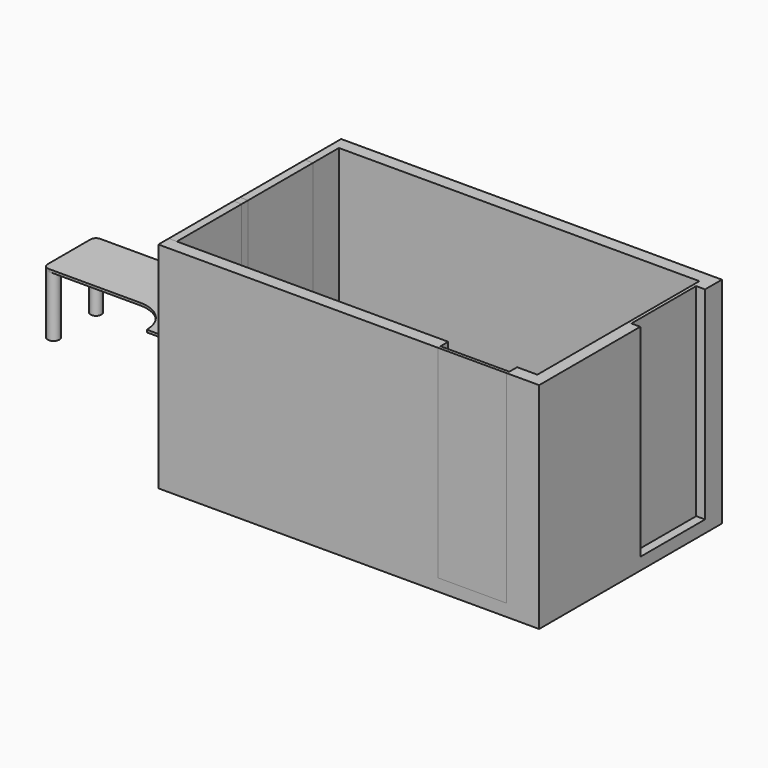
from build123d import *

# Parameters (mm, degrees)
F0_W      = 100
F0_H      = 1000
F0_H_2    = 100
F0_W_2    = 850
F0_H_3    = 120
F0_H_4    = 40
F0_W_3    = 110
F0_W_4    = 40
F1_DEPTH  = 150
F2_DEPTH  = 150
F3_DEPTH  = 2500
F4_DEPTH  = 2500
F5_DEPTH  = 2500
F8_DEPTH  = 15
F9_DEPTH  = 760
F11_W     = 1600
F11_H     = 430
F12_DEPTH = 900
F13_W     = 390
F13_H     = 1450
F14_DEPTH = 770
F15_W     = 322.5
F15_H     = 336
F16_DEPTH = 390
F17_R     = 300
F18_DEPTH = 80
F19_R     = 40
F20_DEPTH = 400
F21_W     = 440
F21_H     = 400
F21_W_2   = 60
F22_DEPTH = 60
F23_DEPTH = 600
F24_R     = 50
F25_SIZE  = 40


with BuildPart() as f1:
    # F0 (on Top) → F1 (new body)
    with BuildSketch(Plane.XY):
        Polygon((300, 2500), (300, 0), (3350, 0), (4200, 0), (4450, 0), (4450, 1400), (4450, 2400), (4450, 2500), align=None)
        Polygon((0, 2500), (300, 2500), (4450, 2500), (4450, 2400), (4490, 2400), (4600, 2400), (4600, 2660), (-100, 2660), (-100, 2100), (0, 2100), align=None)
        with Locations((-50, 1600)):
            Rectangle(F0_W, F0_H)
        with Locations((-50, 1050)):
            Rectangle(F0_W, F0_H_2)
        with Locations((-50, 500)):
            Rectangle(F0_W, F0_H)
        Polygon((300, 0), (0, 0), (-100, 0), (-100, -160), (3350, -160), (3350, -120), (3350, 0), align=None)
        with Locations((3775, -60)):
            Rectangle(F0_W_2, F0_H_3)
        with Locations((3775, -140)):
            Rectangle(F0_W_2, F0_H_4)
        Polygon((4450, 0), (4200, 0), (4200, -120), (4200, -160), (4600, -160), (4600, 1400), (4490, 1400), (4450, 1400), align=None)
        with Locations((4545, 1900)):
            Rectangle(F0_W_3, F0_H)
        with Locations((4470, 1900)):
            Rectangle(F0_W_4, F0_H)
    extrude(amount=-F1_DEPTH)

    # F0 (on Top) → F2 (join, through all)
    with BuildSketch(Plane.XY):
        Polygon((0, 1000), (0, 0), (300, 0), (300, 2500), (0, 2500), (0, 2100), (0, 1100), align=None)
    extrude(amount=-F2_DEPTH)

    # F0 (on Top) → F3 (join)
    with BuildSketch(Plane.XY):
        Polygon((0, 2500), (300, 2500), (4450, 2500), (4450, 2400), (4490, 2400), (4600, 2400), (4600, 2660), (-100, 2660), (-100, 2100), (0, 2100), align=None)
        Polygon((4450, 0), (4200, 0), (4200, -120), (4200, -160), (4600, -160), (4600, 1400), (4490, 1400), (4450, 1400), align=None)
        Polygon((300, 0), (0, 0), (-100, 0), (-100, -160), (3350, -160), (3350, -120), (3350, 0), align=None)
        with Locations((-50, 1050)):
            Rectangle(F0_W, F0_H_2)
    extrude(amount=F3_DEPTH)


with BuildPart() as f4:
    # F0 (on Top) → F4 (new body, through all)
    with BuildSketch(Plane.XY):
        with Locations((-50, 1600)):
            Rectangle(F0_W, F0_H)
    extrude(amount=F4_DEPTH)


with BuildPart() as f4b:
    # F0 (on Top) → F4, piece 2 (new body, through all)
    with BuildSketch(Plane.XY):
        with Locations((-50, 500)):
            Rectangle(F0_W, F0_H)
    extrude(amount=F4_DEPTH)


with BuildPart() as f5:
    # F0 (on Top) → F5 (new body, through all)
    with BuildSketch(Plane.XY):
        with Locations((4470, 1900)):
            Rectangle(F0_W_4, F0_H)
    extrude(amount=F5_DEPTH)


with BuildPart() as f5b:
    # F0 (on Top) → F5, piece 2 (new body, through all)
    with BuildSketch(Plane.XY):
        with Locations((3775, -140)):
            Rectangle(F0_W_2, F0_H_4)
    extrude(amount=F5_DEPTH)


with BuildPart() as f8:
    # F7 (on offset) → F8 (new body, symmetric)
    with BuildSketch(Plane.XY.offset(760)):
        with BuildLine():
            Line((2680.377719402, 2169.4638956216), (646.4488137391, 2169.4638956216))
            ThreePointArc((646.4488137391, 2169.4638956216), (688.5376842462, 2152.0301146325), (705.9714652353, 2109.9412441254))
            ThreePointArc((705.9714652353, 2109.9412441254), (646.4488137391, 2050.4185926292), (586.9261622429, 2109.9412441254))
            Line((586.9261622429, 2109.9412441254), (586.9261622429, 1040.2058445736))
            ThreePointArc((586.9261622429, 1040.2058445736), (657.6681111949, 1110.9477935256), (728.410060147, 1040.2058445736))
            ThreePointArc((728.410060147, 1040.2058445736), (707.6902230133, 990.1837327553), (657.6681111949, 969.4638956216))
            Line((657.6681111949, 969.4638956216), (1146.9261622429, 969.4638956216))
            ThreePointArc((1146.9261622429, 969.4638956216), (1264.0834497683, 1252.3066080962), (1546.9261622429, 1369.4638956216))
            Line((1546.9261622429, 1369.4638956216), (2675.2513630672, 1369.4638956216))
            ThreePointArc((2675.2513630672, 1369.4638956216), (2624.5696265299, 1491.8204313346), (2746.9261622429, 1441.1386947972))
            Line((2746.9261622429, 1441.1386947972), (2746.9261622429, 2102.9154527807))
            ThreePointArc((2746.9261622429, 2102.9154527807), (2633.3208641919, 2055.8585975705), (2680.377719402, 2169.4638956216))
        make_face()
        with BuildLine():
            ThreePointArc((705.9714652353, 2109.9412441254), (688.5376842462, 2152.0301146325), (646.4488137391, 2169.4638956216))
            ThreePointArc((646.4488137391, 2169.4638956216), (604.3599432319, 2152.0301146325), (586.9261622429, 2109.9412441254))
            ThreePointArc((586.9261622429, 2109.9412441254), (646.4488137391, 2050.4185926292), (705.9714652353, 2109.9412441254))
        make_face()
        with BuildLine():
            ThreePointArc((2746.9261622429, 2102.9154527807), (2727.4345746122, 2149.9723079909), (2680.377719402, 2169.4638956216))
            ThreePointArc((2680.377719402, 2169.4638956216), (2633.3208641919, 2055.8585975705), (2746.9261622429, 2102.9154527807))
        make_face()
        with BuildLine():
            ThreePointArc((2675.2513630672, 1369.4638956216), (2725.9330996045, 1390.4569582599), (2746.9261622429, 1441.1386947972))
            ThreePointArc((2746.9261622429, 1441.1386947972), (2624.5696265299, 1491.8204313346), (2675.2513630672, 1369.4638956216))
        make_face()
        with BuildLine():
            ThreePointArc((728.410060147, 1040.2058445736), (657.6681111949, 1110.9477935256), (586.9261622429, 1040.2058445736))
            ThreePointArc((586.9261622429, 1040.2058445736), (607.6459993766, 990.1837327553), (657.6681111949, 969.4638956216))
            ThreePointArc((657.6681111949, 969.4638956216), (707.6902230133, 990.1837327553), (728.410060147, 1040.2058445736))
        make_face()
    extrude(amount=F8_DEPTH, both=True)

    # F7 (on offset) → F9 (join, through all)
    with BuildSketch(Plane.XY.offset(760)):
        with BuildLine():
            ThreePointArc((705.9714652353, 2109.9412441254), (688.5376842462, 2152.0301146325), (646.4488137391, 2169.4638956216))
            ThreePointArc((646.4488137391, 2169.4638956216), (604.3599432319, 2152.0301146325), (586.9261622429, 2109.9412441254))
            ThreePointArc((586.9261622429, 2109.9412441254), (646.4488137391, 2050.4185926292), (705.9714652353, 2109.9412441254))
        make_face()
        with BuildLine():
            ThreePointArc((2746.9261622429, 2102.9154527807), (2727.4345746122, 2149.9723079909), (2680.377719402, 2169.4638956216))
            ThreePointArc((2680.377719402, 2169.4638956216), (2633.3208641919, 2055.8585975705), (2746.9261622429, 2102.9154527807))
        make_face()
        with BuildLine():
            ThreePointArc((2675.2513630672, 1369.4638956216), (2725.9330996045, 1390.4569582599), (2746.9261622429, 1441.1386947972))
            ThreePointArc((2746.9261622429, 1441.1386947972), (2624.5696265299, 1491.8204313346), (2675.2513630672, 1369.4638956216))
        make_face()
        with BuildLine():
            ThreePointArc((728.410060147, 1040.2058445736), (657.6681111949, 1110.9477935256), (586.9261622429, 1040.2058445736))
            ThreePointArc((586.9261622429, 1040.2058445736), (607.6459993766, 990.1837327553), (657.6681111949, 969.4638956216))
            ThreePointArc((657.6681111949, 969.4638956216), (707.6902230133, 990.1837327553), (728.410060147, 1040.2058445736))
        make_face()
    extrude(amount=-F9_DEPTH)


with BuildPart() as f10_1:
    # F10: instance of F8
    add(f8.part.mirror(Plane.YZ))


with BuildPart() as f12:
    # F11 (on Top) → F12 (new body)
    with BuildSketch(Plane.XY):
        with Locations((2296.36054039, 634.8821485043)):
            Rectangle(F11_W, F11_H)
    extrude(amount=F12_DEPTH)


with BuildPart() as f14:
    # F13 (on Top) → F14 (new body)
    with BuildSketch(Plane.XY):
        with Locations((3555.9650611877, 1097.4260926247)):
            Rectangle(F13_W, F13_H)
    extrude(amount=F14_DEPTH)

    # F15 (on face) → F16 (cut, through all)
    with BuildSketch(Plane.YZ.offset(3750.9650611877)):
        with Locations((553.6760926247, 573)):
            Rectangle(F15_W, F15_H)
        with Locations((916.1760926247, 573)):
            Rectangle(F15_W, F15_H)
        with Locations((916.1760926247, 197)):
            Rectangle(F15_W, F15_H)
        with Locations((553.6760926247, 197)):
            Rectangle(F15_W, F15_H)
        with Locations((1278.6760926247, 573)):
            Rectangle(F15_W, F15_H)
        with Locations((1641.1760926247, 573)):
            Rectangle(F15_W, F15_H)
        with Locations((1278.6760926247, 197)):
            Rectangle(F15_W, F15_H)
        with Locations((1641.1760926247, 197)):
            Rectangle(F15_W, F15_H)
    extrude(amount=-F16_DEPTH, mode=Mode.SUBTRACT)


with BuildPart() as f18:
    # F17 (on Top) → F18 (new body)
    with BuildSketch(Plane.XY):
        with Locations((588.9477133751, 499.4027614594)):
            Circle(F17_R)
    extrude(amount=F18_DEPTH)

    # F19 (on face) → F20 (join)
    with BuildSketch(Plane.XY.offset(80)):
        with Locations((588.9477133751, 499.4027614594)):
            Circle(F19_R)
    extrude(amount=F20_DEPTH)

    # F21 (on face) → F22 (join)
    with BuildSketch(Plane.XY.offset(480)):
        with Locations((618.9477133751, 499.4027614594)):
            Rectangle(F21_W, F21_H)
        with Locations((368.9477133751, 499.4027614594)):
            Rectangle(F21_W_2, F21_H)
    extrude(amount=F22_DEPTH)

    # F21 (on face) → F23 (join)
    with BuildSketch(Plane.XY.offset(480)):
        with Locations((368.9477133751, 499.4027614594)):
            Rectangle(F21_W_2, F21_H)
    extrude(amount=F23_DEPTH)

    # F24
    f24_edges = [f18.edges().sort_by_distance(p)[0] for p in [
        (838.947713, 699.402761, 510),
        (838.947713, 299.402761, 510),
        (368.947713, 299.402761, 1080),
        (368.947713, 699.402761, 1080),
    ]]
    fillet(f24_edges, radius=F24_R)

    # F25
    f25_edges = [f18.edges().sort_by_distance(p)[0] for p in [
        (288.947713, 499.402761, 80),
    ]]
    chamfer(f25_edges, length=F25_SIZE)


solid = Compound([f1.part, f4.part, f4b.part, f5.part, f5b.part, f8.part, f10_1.part, f12.part, f14.part, f18.part])
